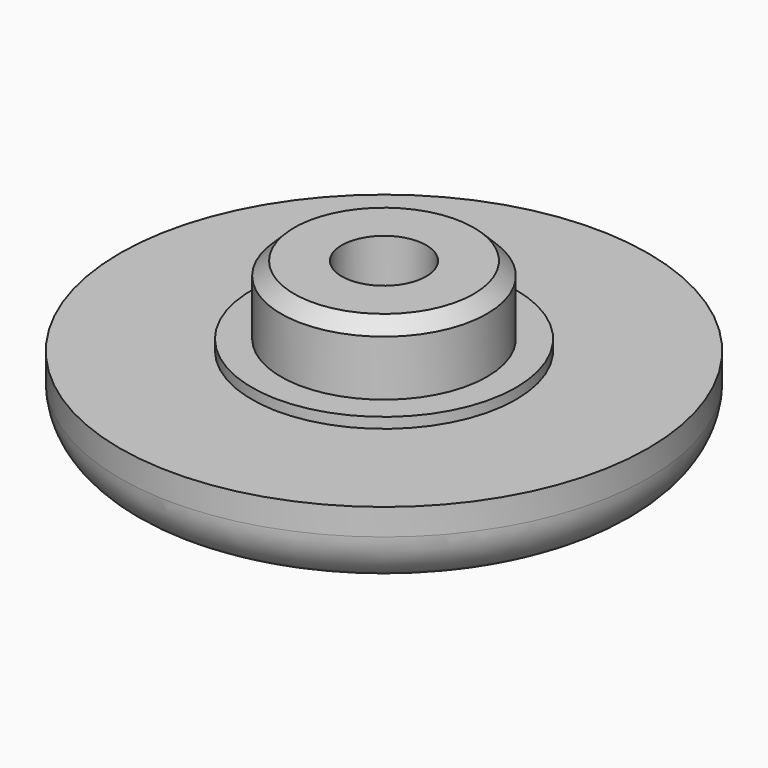
from build123d import *

# Parameters (mm, degrees)
F2_SIZE  = 0.5
F3_R     = 5
F3_R_2   = 3.9
F4_DEPTH = 0.4
F5_R     = 2
F6_R     = 1.6
F7_DEPTH = 25
F8_R     = 3
F8_R_2   = 1.6
F9_DEPTH = 2.5


# Not quite as in the source:
# - a feature names something its author has since deleted; it is built from what else it names


with BuildPart() as f1:
    # F0 (on Front) → F1 (revolve)
    with BuildSketch(Plane.XZ):
        Polygon((3.9, 6), (0, 6), (0, 0), (10, 0), (10, 3), (3.9, 3), align=None)
    revolve(axis=Axis((0, 0, 3), (0, 0, -1)))

    # F2
    f2_edges = [f1.edges().sort_by_distance(p)[0] for p in [
        (-3.9, 0, 6),
    ]]
    chamfer(f2_edges, length=F2_SIZE)

    # F3 (on face) → F4 (join)
    with BuildSketch(Plane.XY.offset(3)):
        Circle(F3_R)
        Circle(F3_R_2, mode=Mode.SUBTRACT)
    extrude(amount=F4_DEPTH)

    # F5
    f5_edges = [f1.edges().sort_by_distance(p)[0] for p in [
        (-10, 0, 0),
    ]]
    fillet(f5_edges, radius=F5_R)

    # F6 (on face) → F7 (cut)
    with BuildSketch(Plane.XY.offset(6)):
        Circle(F6_R)
    extrude(amount=-F7_DEPTH, mode=Mode.SUBTRACT)

    # F8 (on face) → F9 (cut)
    with BuildSketch(Plane(origin=(0, 0, 0), x_dir=(1, 0, 0), z_dir=(0, 0, -1))):
        Circle(F8_R)
        Circle(F8_R_2, mode=Mode.SUBTRACT)
    extrude(amount=-F9_DEPTH, mode=Mode.SUBTRACT)


solid = f1.part
